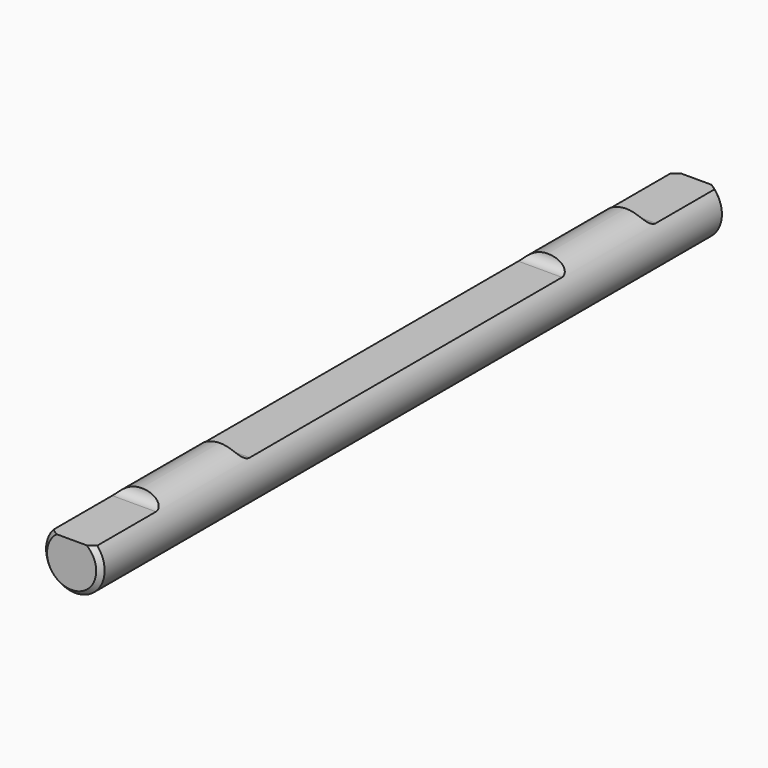
from build123d import *

# Parameters (mm, degrees)
F0_R     = 9.525
F1_DEPTH = 127
F2_W     = 133.35
F2_H     = 3.175
F2_W_2   = 28.575
F3_DEPTH = 12.7
F4_SIZE  = 1.524
F5_R     = 3.17499


# Not quite as in the source:
# - a fillet or chamfer is up to 0.001 mm smaller than in the source, because OpenCascade refuses the exact size


with BuildPart() as f1:
    # F0 (on Front) → F1 (new body, symmetric)
    with BuildSketch(Plane.XZ):
        Circle(F0_R)
    extrude(amount=F1_DEPTH, both=True)

    # F2 (on Right) → F3 (cut, symmetric)
    with BuildSketch(Plane.YZ):
        with Locations((0, 7.9375)):
            Rectangle(F2_W, F2_H)
        with Locations((-112.7125, 7.9375)):
            Rectangle(F2_W_2, F2_H)
        with Locations((112.7125, 7.9375)):
            Rectangle(F2_W_2, F2_H)
    extrude(amount=F3_DEPTH, both=True, mode=Mode.SUBTRACT)

    # F4
    f4_edges = [f1.edges().sort_by_distance(p)[0] for p in [
        (-3.39873, -127, -8.897992),
        (-3.39873, 127, -8.897992),
    ]]
    chamfer(f4_edges, length=F4_SIZE)

    # F5 (radius 3.175 in the source; OpenCascade refuses exactly that, so slightly less here)
    f5_edges = [f1.edges().sort_by_distance(p)[0] for p in [
        (0, -98.425, 6.35),
        (0, 66.675, 6.35),
        (0, 98.425, 6.35),
        (0, -66.675, 6.35),
    ]]
    fillet(f5_edges, radius=F5_R)


solid = f1.part
